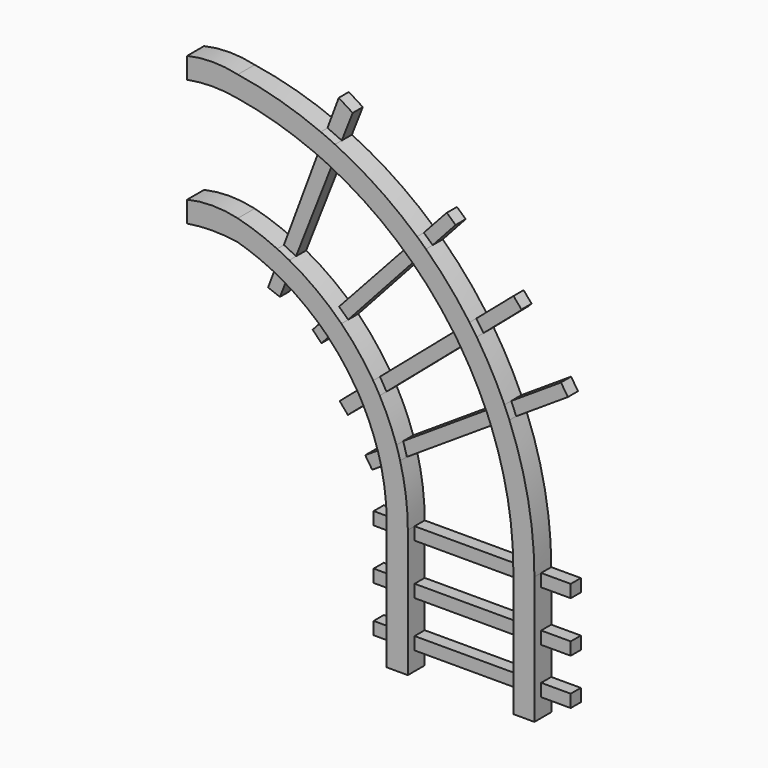
from build123d import *

# Parameters (mm, degrees)
F0_W     = 12.7
F0_H     = 7.62
F0_H_2   = 22.86
F0_H_3   = 20.1060211349
F0_H_4   = 11.0575035214
F1_DEPTH = 12.7
F2_DEPTH = 7.62
F0_W_2   = 11.9574208686
F0_W_3   = 63.5
F0_W_4   = 17.7985066107


# Not quite as in the source:
# - a feature names something its author has since deleted; it is built from what else it names


with BuildPart() as f1:
    # F0 (on Front) → F1 (new body)
    with BuildSketch(Plane.XZ):
        with BuildLine():
            ThreePointArc((-124.2340589469, 111.8650491221), (-120.6911886684, 110.0883004357), (-117.2068306171, 108.1993815187))
            Line((-117.2068306171, 108.1993815187), (-112.6487632581, 119.831367092))
            ThreePointArc((-112.6487632581, 119.831367092), (-116.2533464719, 121.7134549995), (-119.9124850246, 123.4871460914))
            Line((-119.9124850246, 123.4871460914), (-124.2340589469, 111.8650491221))
        make_face()
        with BuildLine():
            ThreePointArc((-117.2068306171, 108.1993815187), (-105.7437326029, 100.892298193), (-95.1481311046, 92.3758839417))
            Line((-95.1481311046, 92.3758839417), (-86.7118367758, 101.5981585056))
            ThreePointArc((-86.7118367758, 101.5981585056), (-99.1481868245, 111.4716992803), (-112.6487632581, 119.831367092))
            Line((-112.6487632581, 119.831367092), (-117.2068306171, 108.1993815187))
        make_face()
        with BuildLine():
            ThreePointArc((-95.1481311046, 92.3758839417), (-92.3730160909, 89.8059248015), (-89.6774651275, 87.1526328225))
            Line((-89.6774651275, 87.1526328225), (-81.249594387, 96.4386708505))
            ThreePointArc((-81.249594387, 96.4386708505), (-83.9451451597, 99.0560723446), (-86.7118367758, 101.5981585056))
            Line((-86.7118367758, 101.5981585056), (-95.1481311046, 92.3758839417))
        make_face()
        with BuildLine():
            ThreePointArc((-89.6774651275, 87.1526328225), (-80.0673386841, 76.1799771384), (-71.8102795189, 64.1560561074))
            Line((-71.8102795189, 64.1560561074), (-62.1175916172, 72.4640760933))
            ThreePointArc((-62.1175916172, 72.4640760933), (-71.0068424868, 84.9914281783), (-81.249594387, 96.4386708505))
            Line((-81.249594387, 96.4386708505), (-89.6774651275, 87.1526328225))
        make_face()
        with BuildLine():
            ThreePointArc((-71.8102795189, 64.1560561074), (-69.8549191799, 60.7983440342), (-68.0055774583, 57.3810937335))
            Line((-68.0055774583, 57.3810937335), (-58.1892259059, 65.7951091971))
            ThreePointArc((-58.1892259059, 65.7951091971), (-60.1060468891, 69.1574912326), (-62.1175916172, 72.4640760933))
            Line((-62.1175916172, 72.4640760933), (-71.8102795189, 64.1560561074))
        make_face()
        with BuildLine():
            ThreePointArc((-68.0055774583, 57.3810937335), (-63.0811522272, 46.7318419885), (-59.1838581618, 35.665332803))
            Line((-59.1838581618, 35.665332803), (-48.1652278842, 42.8527283219))
            ThreePointArc((-48.1652278842, 42.8527283219), (-52.6491743747, 54.5546357652), (-58.1892259059, 65.7951091971))
            Line((-58.1892259059, 65.7951091971), (-68.0055774583, 57.3810937335))
        make_face()
        with BuildLine():
            ThreePointArc((-59.1838581618, 35.665332803), (-58.0934616874, 31.8034206446), (-57.1284306901, 27.9082896886))
            Line((-57.1284306901, 27.9082896886), (-45.8873909346, 35.2407617592))
            ThreePointArc((-45.8873909346, 35.2407617592), (-46.9708146032, 39.0633515402), (-48.1652278842, 42.8527283219))
            Line((-48.1652278842, 42.8527283219), (-59.1838581618, 35.665332803))
        make_face()
        with BuildLine():
            ThreePointArc((-57.1284306901, 27.9082896886), (-54.7481910079, 14.0442724608), (-53.9513687661, 0))
            Line((-53.9513687661, 0), (-41.2513687661, 0))
            ThreePointArc((-41.2513687661, 0), (-42.4153458619, 17.7721973242), (-45.8873909346, 35.2407617592))
            Line((-45.8873909346, 35.2407617592), (-57.1284306901, 27.9082896886))
        make_face()
        with Locations((-47.6013687661, -3.81)):
            Rectangle(F0_W, F0_H)
        with Locations((-47.6013687661, -19.05)):
            Rectangle(F0_W, F0_H_2)
        with Locations((-47.6013687661, -34.29)):
            Rectangle(F0_W, F0_H)
        with Locations((-47.6013687661, -48.1530105674)):
            Rectangle(F0_W, F0_H_3)
        with Locations((-47.6013687661, -62.0160211349)):
            Rectangle(F0_W, F0_H)
        with Locations((-47.6013687661, -71.3547728956)):
            Rectangle(F0_W, F0_H_4)
        with BuildLine():
            ThreePointArc((-143.6181953794, 119.2770247535), (-133.7710028536, 115.9767251012), (-124.2340589469, 111.8650491221))
            Line((-124.2340589469, 111.8650491221), (-119.9124850246, 123.4871460914))
            ThreePointArc((-119.9124850246, 123.4871460914), (-131.5688085246, 128.280847449), (-143.6181953794, 131.9770247535))
            ThreePointArc((-143.6181953794, 131.9770247535), (-158.8594909135, 133.7390513428), (-174.1007864475, 131.9770247535))
            Line((-174.1007864475, 131.9770247535), (-174.1007864475, 119.2770247535))
            ThreePointArc((-174.1007864475, 119.2770247535), (-158.8594909135, 120.514270152), (-143.6181953794, 119.2770247535))
        make_face()
    extrude(amount=F1_DEPTH)


with BuildPart() as f1b:
    # F0 (on Front) → F1, piece 2 (new body)
    with BuildSketch(Plane.XZ):
        with Locations((28.5986312339, -71.3547728956)):
            Rectangle(F0_W, F0_H_4)
        with Locations((28.5986312339, -62.0160211349)):
            Rectangle(F0_W, F0_H)
        with Locations((28.5986312339, -48.1530105674)):
            Rectangle(F0_W, F0_H_3)
        with Locations((28.5986312339, -34.29)):
            Rectangle(F0_W, F0_H)
        with Locations((28.5986312339, -19.05)):
            Rectangle(F0_W, F0_H_2)
        with Locations((28.5986312339, -3.81)):
            Rectangle(F0_W, F0_H)
        with BuildLine():
            ThreePointArc((9.0582243895, 71.0815023427), (18.9231196005, 36.1474992497), (22.2486312339, 0))
            Line((22.2486312339, 0), (34.9486312339, 0))
            ThreePointArc((34.9486312339, 0), (31.1548479697, 39.7968808399), (19.9101610736, 78.1601644931))
            Line((19.9101610736, 78.1601644931), (9.0582243895, 71.0815023427))
        make_face()
        with BuildLine():
            ThreePointArc((6.1320695683, 78.2705745122), (7.6303562647, 74.6903695983), (9.0582243895, 71.0815023427))
            Line((9.0582243895, 71.0815023427), (19.9101610736, 78.1601644931))
            ThreePointArc((19.9101610736, 78.1601644931), (18.440247544, 81.7426565391), (16.9047235594, 85.2975209721))
            Line((16.9047235594, 85.2975209721), (6.1320695683, 78.2705745122))
        make_face()
        with BuildLine():
            ThreePointArc((-9.4812919147, 107.544766146), (-1.0607428596, 93.2350763939), (6.1320695683, 78.2705745122))
            Line((6.1320695683, 78.2705745122), (16.9047235594, 85.2975209721))
            ThreePointArc((16.9047235594, 85.2975209721), (9.1952524724, 100.9244084009), (0.2204899498, 115.8605790217))
            Line((0.2204899498, 115.8605790217), (-9.4812919147, 107.544766146))
        make_face()
        with BuildLine():
            ThreePointArc((-13.7693080337, 113.9054709235), (-11.5945117384, 110.7458741674), (-9.4812919147, 107.544766146))
            Line((-9.4812919147, 107.544766146), (0.2204899498, 115.8605790217))
            ThreePointArc((0.2204899498, 115.8605790217), (-1.9166461977, 119.0418729884), (-4.1113104413, 122.1837563524))
            Line((-4.1113104413, 122.1837563524), (-13.7693080337, 113.9054709235))
        make_face()
        with BuildLine():
            ThreePointArc((-38.8785813269, 143.124109044), (-25.6120454144, 129.1265663831), (-13.7693080337, 113.9054709235))
            Line((-13.7693080337, 113.9054709235), (-4.1113104413, 122.1837563524))
            ThreePointArc((-4.1113104413, 122.1837563524), (-16.5226225014, 137.9626725851), (-30.3797347969, 152.4883499656))
            Line((-30.3797347969, 152.4883499656), (-38.8785813269, 143.124109044))
        make_face()
        with BuildLine():
            ThreePointArc((-44.2182951371, 148.0506757973), (-41.5258536483, 145.6118709712), (-38.8785813269, 143.124109044))
            Line((-38.8785813269, 143.124109044), (-30.3797347969, 152.4883499656))
            ThreePointArc((-30.3797347969, 152.4883499656), (-33.0129166599, 154.9547842327), (-35.6879580546, 157.3757547516))
            Line((-35.6879580546, 157.3757547516), (-44.2182951371, 148.0506757973))
        make_face()
        with BuildLine():
            ThreePointArc((-89.6990374912, 178.3980485394), (-65.9067493948, 164.8008400662), (-44.2182951371, 148.0506757973))
            Line((-44.2182951371, 148.0506757973), (-35.6879580546, 157.3757547516))
            ThreePointArc((-35.6879580546, 157.3757547516), (-59.2307929883, 175.5125125411), (-85.0918920618, 190.1552791699))
            Line((-85.0918920618, 190.1552791699), (-89.6990374912, 178.3980485394))
        make_face()
        with BuildLine():
            ThreePointArc((-98.0777279488, 182.2078040271), (-93.8662557532, 180.3515895127), (-89.6990374912, 178.3980485394))
            Line((-89.6990374912, 178.3980485394), (-85.0918920618, 190.1552791699))
            ThreePointArc((-85.0918920618, 190.1552791699), (-89.3677361828, 192.1339575614), (-93.6867674836, 194.0165036426))
            Line((-93.6867674836, 194.0165036426), (-98.0777279488, 182.2078040271))
        make_face()
        with BuildLine():
            ThreePointArc((-143.6181953794, 195.4770247535), (-120.44941117, 190.2102547609), (-98.0777279488, 182.2078040271))
            Line((-98.0777279488, 182.2078040271), (-93.6867674836, 194.0165036426))
            ThreePointArc((-93.6867674836, 194.0165036426), (-118.2146627055, 202.6405572531), (-143.6181953794, 208.1770247535))
            ThreePointArc((-143.6181953794, 208.1770247535), (-158.8594909135, 209.932990889), (-174.1007864475, 208.1770247535))
            Line((-174.1007864475, 208.1770247535), (-174.1007864475, 195.4770247535))
            ThreePointArc((-174.1007864475, 195.4770247535), (-158.8594909135, 196.9287437083), (-143.6181953794, 195.4770247535))
        make_face()
    extrude(amount=F1_DEPTH)


with BuildPart() as f2:
    # F0 (on Front) → F2 (new body)
    with BuildSketch(Plane.XZ):
        with BuildLine():
            Line((-122.3074973381, 95.1827064589), (-117.2068306171, 108.1993815187))
            ThreePointArc((-117.2068306171, 108.1993815187), (-120.6911886684, 110.0883004357), (-124.2340589469, 111.8650491221))
            Line((-124.2340589469, 111.8650491221), (-129.4497156294, 97.8384771341))
            Line((-129.4497156294, 97.8384771341), (-122.3074973381, 95.1827064589))
        make_face()
    extrude(amount=F2_DEPTH)


with BuildPart() as f2b:
    # F0 (on Front) → F2, piece 2 (new body)
    with BuildSketch(Plane.XZ):
        with BuildLine():
            ThreePointArc((-119.9124850246, 123.4871460914), (-116.2533464719, 121.7134549995), (-112.6487632581, 119.831367092))
            Line((-112.6487632581, 119.831367092), (-89.6990374912, 178.3980485394))
            ThreePointArc((-89.6990374912, 178.3980485394), (-93.8662557532, 180.3515895127), (-98.0777279488, 182.2078040271))
            Line((-98.0777279488, 182.2078040271), (-119.9124850246, 123.4871460914))
        make_face()
    extrude(amount=F2_DEPTH)


with BuildPart() as f2c:
    # F0 (on Front) → F2, piece 3 (new body)
    with BuildSketch(Plane.XZ):
        with BuildLine():
            ThreePointArc((-93.6867674836, 194.0165036426), (-89.3677361828, 192.1339575614), (-85.0918920618, 190.1552791699))
            Line((-85.0918920618, 190.1552791699), (-78.5144492984, 206.9406211376))
            Line((-78.5144492984, 206.9406211376), (-86.9173908385, 212.2215264434))
            Line((-86.9173908385, 212.2215264434), (-93.6867674836, 194.0165036426))
        make_face()
    extrude(amount=F2_DEPTH)


with BuildPart() as f2d:
    # F0 (on Front) → F2, piece 4 (new body)
    with BuildSketch(Plane.XZ):
        with BuildLine():
            ThreePointArc((-35.6879580546, 157.3757547516), (-33.0129166599, 154.9547842327), (-30.3797347969, 152.4883499656))
            Line((-30.3797347969, 152.4883499656), (-16.5886765187, 167.6836816882))
            Line((-16.5886765187, 167.6836816882), (-21.809151895, 172.4592353225))
            Line((-21.809151895, 172.4592353225), (-22.9627117515, 171.2865680456))
            Line((-22.9627117515, 171.2865680456), (-35.6879580546, 157.3757547516))
        make_face()
    extrude(amount=F2_DEPTH)


with BuildPart() as f2e:
    # F0 (on Front) → F2, piece 5 (new body)
    with BuildSketch(Plane.XZ):
        with BuildLine():
            ThreePointArc((-86.7118367758, 101.5981585056), (-83.9451451597, 99.0560723446), (-81.249594387, 96.4386708505))
            Line((-81.249594387, 96.4386708505), (-38.8785813269, 143.124109044))
            ThreePointArc((-38.8785813269, 143.124109044), (-41.5258536483, 145.6118709712), (-44.2182951371, 148.0506757973))
            Line((-44.2182951371, 148.0506757973), (-86.7118367758, 101.5981585056))
        make_face()
    extrude(amount=F2_DEPTH)


with BuildPart() as f2f:
    # F0 (on Front) → F2, piece 6 (new body)
    with BuildSketch(Plane.XZ):
        with BuildLine():
            Line((-97.311937048, 78.7407813882), (-89.6774651275, 87.1526328225))
            ThreePointArc((-89.6774651275, 87.1526328225), (-92.3730160909, 89.8059248015), (-95.1481311046, 92.3758839417))
            Line((-95.1481311046, 92.3758839417), (-102.6202812791, 84.2075794935))
            Line((-102.6202812791, 84.2075794935), (-97.311937048, 78.7407813882))
        make_face()
    extrude(amount=F2_DEPTH)


with BuildPart() as f2g:
    # F0 (on Front) → F2, piece 7 (new body)
    with BuildSketch(Plane.XZ):
        with BuildLine():
            Line((-81.4049914479, 45.8958819509), (-68.0055774583, 57.3810937335))
            ThreePointArc((-68.0055774583, 57.3810937335), (-69.8549191799, 60.7983440342), (-71.8102795189, 64.1560561074))
            Line((-71.8102795189, 64.1560561074), (-86.3640223277, 51.6814167346))
            Line((-86.3640223277, 51.6814167346), (-81.4049914479, 45.8958819509))
        make_face()
    extrude(amount=F2_DEPTH)


with BuildPart() as f2h:
    # F0 (on Front) → F2, piece 8 (new body)
    with BuildSketch(Plane.XZ):
        with BuildLine():
            ThreePointArc((-62.1175916172, 72.4640760933), (-60.1060468891, 69.1574912326), (-58.1892259059, 65.7951091971))
            Line((-58.1892259059, 65.7951091971), (-9.4812919147, 107.544766146))
            ThreePointArc((-9.4812919147, 107.544766146), (-11.5945117384, 110.7458741674), (-13.7693080337, 113.9054709235))
            Line((-13.7693080337, 113.9054709235), (-62.1175916172, 72.4640760933))
        make_face()
    extrude(amount=F2_DEPTH)


with BuildPart() as f2i:
    # F0 (on Front) → F2, piece 9 (new body)
    with BuildSketch(Plane.XZ):
        with BuildLine():
            ThreePointArc((-4.1113104413, 122.1837563524), (-1.9166461977, 119.0418729884), (0.2204899498, 115.8605790217))
            Line((0.2204899498, 115.8605790217), (21.2094094604, 133.8510811329))
            Line((21.2094094604, 133.8510811329), (23.1081575649, 135.799651649))
            Line((23.1081575649, 135.799651649), (18.3077638043, 141.4001098334))
            Line((18.3077638043, 141.4001098334), (-4.1113104413, 122.1837563524))
        make_face()
    extrude(amount=F2_DEPTH)


with BuildPart() as f2j:
    # F0 (on Front) → F2, piece 10 (new body)
    with BuildSketch(Plane.XZ):
        with BuildLine():
            ThreePointArc((16.9047235594, 85.2975209721), (18.440247544, 81.7426565391), (19.9101610736, 78.1601644931))
            Line((19.9101610736, 78.1601644931), (51.0417576753, 98.4671438793))
            Line((51.0417576753, 98.4671438793), (46.8786656857, 104.8493683338))
            Line((46.8786656857, 104.8493683338), (16.9047235594, 85.2975209721))
        make_face()
    extrude(amount=F2_DEPTH)


with BuildPart() as f2k:
    # F0 (on Front) → F2, piece 11 (new body)
    with BuildSketch(Plane.XZ):
        with BuildLine():
            ThreePointArc((-48.1652278842, 42.8527283219), (-46.9708146032, 39.0633515402), (-45.8873909346, 35.2407617592))
            Line((-45.8873909346, 35.2407617592), (9.0582243895, 71.0815023427))
            ThreePointArc((9.0582243895, 71.0815023427), (7.6303562647, 74.6903695983), (6.1320695683, 78.2705745122))
            Line((6.1320695683, 78.2705745122), (-48.1652278842, 42.8527283219))
        make_face()
    extrude(amount=F2_DEPTH)


with BuildPart() as f2l:
    # F0 (on Front) → F2, piece 12 (new body)
    with BuildSketch(Plane.XZ):
        with BuildLine():
            Line((-66.7693415597, 21.6195734111), (-57.1284306901, 27.9082896886))
            ThreePointArc((-57.1284306901, 27.9082896886), (-58.0934616874, 31.8034206446), (-59.1838581618, 35.665332803))
            Line((-59.1838581618, 35.665332803), (-70.9463506937, 27.9927197844))
            Line((-70.9463506937, 27.9927197844), (-66.7693415597, 21.6195734111))
        make_face()
    extrude(amount=F2_DEPTH)


with BuildPart() as f2m:
    # F0 (on Front) → F2, piece 13 (new body)
    with BuildSketch(Plane.XZ):
        with Locations((-59.9300792004, -3.81)):
            Rectangle(F0_W_2, F0_H)
    extrude(amount=F2_DEPTH)


with BuildPart() as f2n:
    # F0 (on Front) → F2, piece 14 (new body)
    with BuildSketch(Plane.XZ):
        with Locations((-59.9300792004, -34.29)):
            Rectangle(F0_W_2, F0_H)
    extrude(amount=F2_DEPTH)


with BuildPart() as f2o:
    # F0 (on Front) → F2, piece 15 (new body)
    with BuildSketch(Plane.XZ):
        with Locations((-59.9300792004, -62.0160211349)):
            Rectangle(F0_W_2, F0_H)
    extrude(amount=F2_DEPTH)


with BuildPart() as f2p:
    # F0 (on Front) → F2, piece 16 (new body)
    with BuildSketch(Plane.XZ):
        with Locations((-9.5013687661, -62.0160211349)):
            Rectangle(F0_W_3, F0_H)
    extrude(amount=F2_DEPTH)


with BuildPart() as f2q:
    # F0 (on Front) → F2, piece 17 (new body)
    with BuildSketch(Plane.XZ):
        with Locations((-9.5013687661, -34.29)):
            Rectangle(F0_W_3, F0_H)
    extrude(amount=F2_DEPTH)


with BuildPart() as f2r:
    # F0 (on Front) → F2, piece 18 (new body)
    with BuildSketch(Plane.XZ):
        with Locations((-9.5013687661, -3.81)):
            Rectangle(F0_W_3, F0_H)
    extrude(amount=F2_DEPTH)


with BuildPart() as f2s:
    # F0 (on Front) → F2, piece 19 (new body)
    with BuildSketch(Plane.XZ):
        with Locations((43.8478845392, -3.81)):
            Rectangle(F0_W_4, F0_H)
    extrude(amount=F2_DEPTH)


with BuildPart() as f2t:
    # F0 (on Front) → F2, piece 20 (new body)
    with BuildSketch(Plane.XZ):
        with Locations((43.8478845392, -34.29)):
            Rectangle(F0_W_4, F0_H)
    extrude(amount=F2_DEPTH)


with BuildPart() as f2u:
    # F0 (on Front) → F2, piece 21 (new body)
    with BuildSketch(Plane.XZ):
        with Locations((43.8478845392, -62.0160211349)):
            Rectangle(F0_W_4, F0_H)
    extrude(amount=F2_DEPTH)


solid = Compound([f1.part, f1b.part, f2.part, f2b.part, f2c.part, f2d.part, f2e.part, f2f.part, f2g.part, f2h.part, f2i.part, f2j.part, f2k.part, f2l.part, f2m.part, f2n.part, f2o.part, f2p.part, f2q.part, f2r.part, f2s.part, f2t.part, f2u.part])
